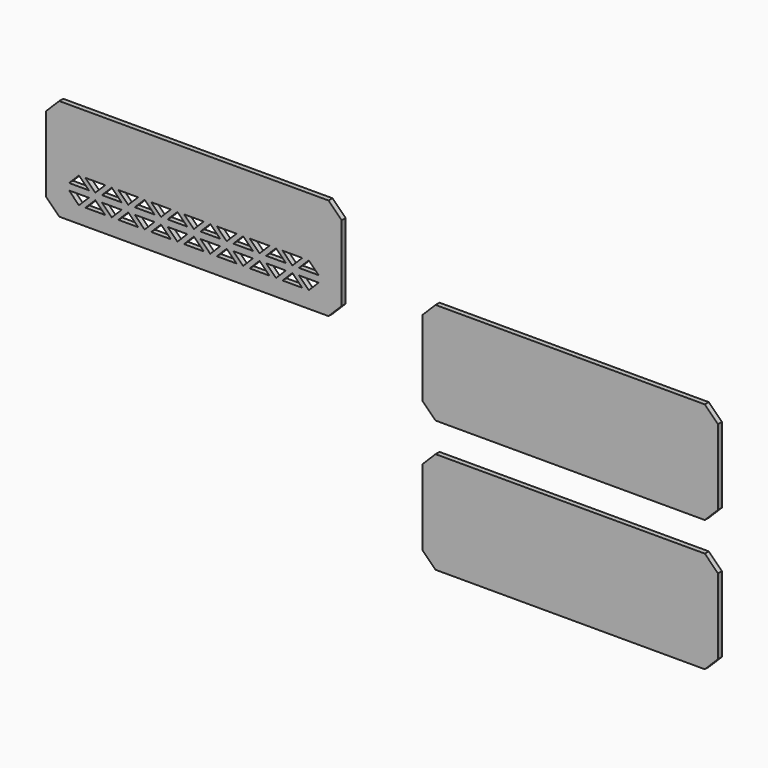
from build123d import *

# Parameters (mm, degrees)
F0_W     = 180
F0_H     = 62
F1_DEPTH = 3
F2_SIZE  = 8
F4_DEPTH = 25
F5_W     = 180
F5_H     = 62
F6_DEPTH = 3
F7_SIZE  = 8


with BuildPart() as f1:
    # F0 (on Front) → F1 (new body)
    with BuildSketch(Plane.XZ):
        with Locations((-229.1829290857, 34.7874979898)):
            Rectangle(F0_W, F0_H)
    extrude(amount=F1_DEPTH)

    # F2
    f2_edges = [f1.edges().sort_by_distance(p)[0] for p in [
        (-319.182929, -1.5, 65.787498),
        (-319.182929, -1.5, 3.787498),
        (-139.182929, -1.5, 3.787498),
        (-139.182929, -1.5, 65.787498),
    ]]
    chamfer(f2_edges, length=F2_SIZE)

    # F3 (on face) → F4 (cut)
    with BuildSketch(Plane.XZ.offset(3)):
        Polygon((-293.1829290857, 19.7874979898), (-305.1829290857, 19.7874979898), (-299.1829290857, 13.7874979898), align=None)
        Polygon((-283.1829290857, 13.7874979898), (-289.1829290857, 19.7874979898), (-295.1829290857, 13.7874979898), align=None)
        Polygon((-275.1829290857, 13.7874979898), (-263.1829290857, 13.7874979898), (-269.1829290857, 19.7874979898), align=None)
        Polygon((-273.1829290857, 19.7874979898), (-285.1829290857, 19.7874979898), (-279.1829290857, 13.7874979898), align=None)
        Polygon((-255.1829290857, 13.7874979898), (-243.1829290857, 13.7874979898), (-249.1829290857, 19.7874979898), align=None)
        Polygon((-253.1829290857, 19.7874979898), (-265.1829290857, 19.7874979898), (-259.1829290857, 13.7874979898), align=None)
        Polygon((-235.1829290857, 13.7874979898), (-223.1829290857, 13.7874979898), (-229.1829290857, 19.7874979898), align=None)
        Polygon((-233.1829290857, 19.7874979898), (-245.1829290857, 19.7874979898), (-239.1829290857, 13.7874979898), align=None)
        Polygon((-215.1829290857, 13.7874979898), (-203.1829290857, 13.7874979898), (-209.1829290857, 19.7874979898), align=None)
        Polygon((-213.1829290857, 19.7874979898), (-225.1829290857, 19.7874979898), (-219.1829290857, 13.7874979898), align=None)
        Polygon((-195.1829290857, 13.7874979898), (-183.1829290857, 13.7874979898), (-189.1829290857, 19.7874979898), align=None)
        Polygon((-193.1829290857, 19.7874979898), (-205.1829290857, 19.7874979898), (-199.1829290857, 13.7874979898), align=None)
        Polygon((-175.1829290857, 13.7874979898), (-163.1829290857, 13.7874979898), (-169.1829290857, 19.7874979898), align=None)
        Polygon((-173.1829290857, 19.7874979898), (-185.1829290857, 19.7874979898), (-179.1829290857, 13.7874979898), align=None)
        Polygon((-299.1829290857, 29.7874979898), (-305.1829290857, 23.7874979898), (-293.1829290857, 23.7874979898), align=None)
        Polygon((-295.1829290857, 29.7874979898), (-289.1829290857, 23.7874979898), (-283.1829290857, 29.7874979898), align=None)
        Polygon((-263.1829290857, 29.7874979898), (-275.1829290857, 29.7874979898), (-269.1829290857, 23.7874979898), align=None)
        Polygon((-279.1829290857, 29.7874979898), (-285.1829290857, 23.7874979898), (-273.1829290857, 23.7874979898), align=None)
        Polygon((-243.1829290857, 29.7874979898), (-255.1829290857, 29.7874979898), (-249.1829290857, 23.7874979898), align=None)
        Polygon((-259.1829290857, 29.7874979898), (-265.1829290857, 23.7874979898), (-253.1829290857, 23.7874979898), align=None)
        Polygon((-223.1829290857, 29.7874979898), (-235.1829290857, 29.7874979898), (-229.1829290857, 23.7874979898), align=None)
        Polygon((-239.1829290857, 29.7874979898), (-245.1829290857, 23.7874979898), (-233.1829290857, 23.7874979898), align=None)
        Polygon((-203.1829290857, 29.7874979898), (-215.1829290857, 29.7874979898), (-209.1829290857, 23.7874979898), align=None)
        Polygon((-219.1829290857, 29.7874979898), (-225.1829290857, 23.7874979898), (-213.1829290857, 23.7874979898), align=None)
        Polygon((-183.1829290857, 29.7874979898), (-195.1829290857, 29.7874979898), (-189.1829290857, 23.7874979898), align=None)
        Polygon((-199.1829290857, 29.7874979898), (-205.1829290857, 23.7874979898), (-193.1829290857, 23.7874979898), align=None)
        Polygon((-163.1829290857, 29.7874979898), (-175.1829290857, 29.7874979898), (-169.1829290857, 23.7874979898), align=None)
        Polygon((-179.1829290857, 29.7874979898), (-185.1829290857, 23.7874979898), (-173.1829290857, 23.7874979898), align=None)
        Polygon((-165.1829290857, 19.7874979898), (-159.1829290857, 13.7874979898), (-153.1829290857, 19.7874979898), align=None)
        Polygon((-153.1829290857, 23.7874979898), (-159.1829290857, 29.7874979898), (-165.1829290857, 23.7874979898), align=None)
    extrude(amount=-F4_DEPTH, mode=Mode.SUBTRACT)


with BuildPart() as f6:
    # F5 (on Front) → F6 (new body)
    with BuildSketch(Plane.XZ):
        Rectangle(F5_W, F5_H)
    extrude(amount=F6_DEPTH)

    # F7
    f7_edges = [f6.edges().sort_by_distance(p)[0] for p in [
        (-90, -1.5, -31),
        (-90, -1.5, 31),
        (90, -1.5, 31),
        (90, -1.5, -31),
    ]]
    chamfer(f7_edges, length=F7_SIZE)


with BuildPart() as f8_1:
    # F8: copy of F6
    add(f6.part.moved(Location((0, 0, -80))))


solid = Compound([f1.part, f6.part, f8_1.part])
